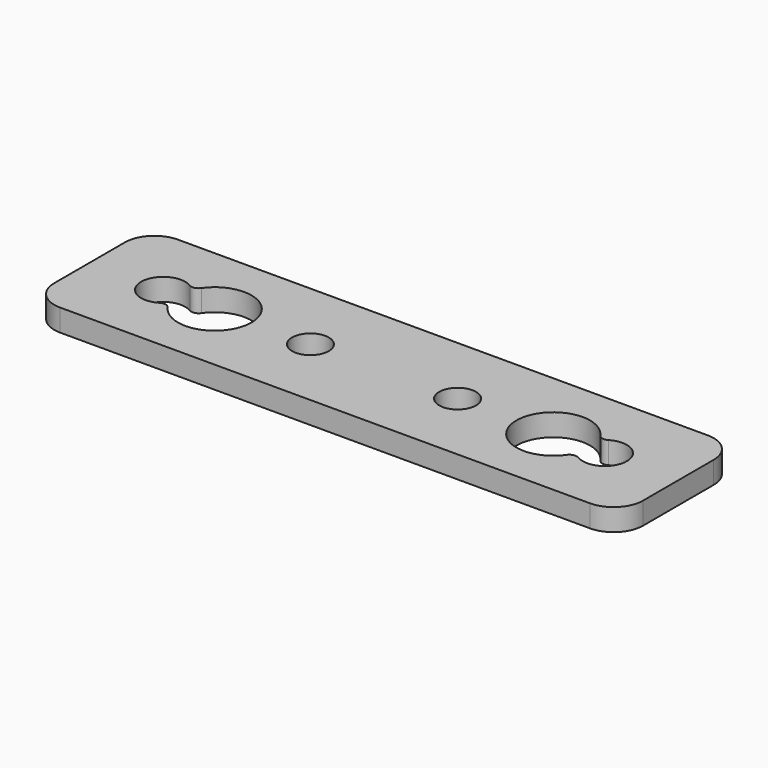
from build123d import *

# Parameters (mm, degrees)
F0_W     = 101.6
F0_H     = 25.4
F0_R     = 3.175
F1_DEPTH = 3.81
F2_R     = 1.27
F3_R     = 5.08


with BuildPart() as f1:
    # F0 (on Top) → F1 (new body)
    with BuildSketch(Plane.XY):
        Rectangle(F0_W, F0_H)
        with BuildLine():
            ThreePointArc((-35.1064285714, 2.3568262774), (-22.86, 0), (-35.1064285714, -2.3568262774))
            ThreePointArc((-35.1064285714, -2.3568262774), (-41.91, 0), (-35.1064285714, 2.3568262774))
        make_face(mode=Mode.SUBTRACT)
        with Locations((-12.7, 0)):
            Circle(F0_R, mode=Mode.SUBTRACT)
        with Locations((12.7, 0)):
            Circle(F0_R, mode=Mode.SUBTRACT)
        with BuildLine():
            ThreePointArc((35.1064285714, -2.3568262774), (22.86, 0), (35.1064285714, 2.3568262774))
            ThreePointArc((35.1064285714, 2.3568262774), (41.91, 0), (35.1064285714, -2.3568262774))
        make_face(mode=Mode.SUBTRACT)
    extrude(amount=F1_DEPTH)

    # F2
    f2_edges = [f1.edges().sort_by_distance(p)[0] for p in [
        (-35.106429, -2.356826, 1.905),
        (35.106429, 2.356826, 1.905),
        (-35.106429, 2.356826, 1.905),
        (35.106429, -2.356826, 1.905),
    ]]
    fillet(f2_edges, radius=F2_R)

    # F3
    f3_edges = [f1.edges().sort_by_distance(p)[0] for p in [
        (-50.8, 12.7, 1.905),
        (-50.8, -12.7, 1.905),
        (50.8, -12.7, 1.905),
        (50.8, 12.7, 1.905),
    ]]
    fillet(f3_edges, radius=F3_R)


solid = f1.part
